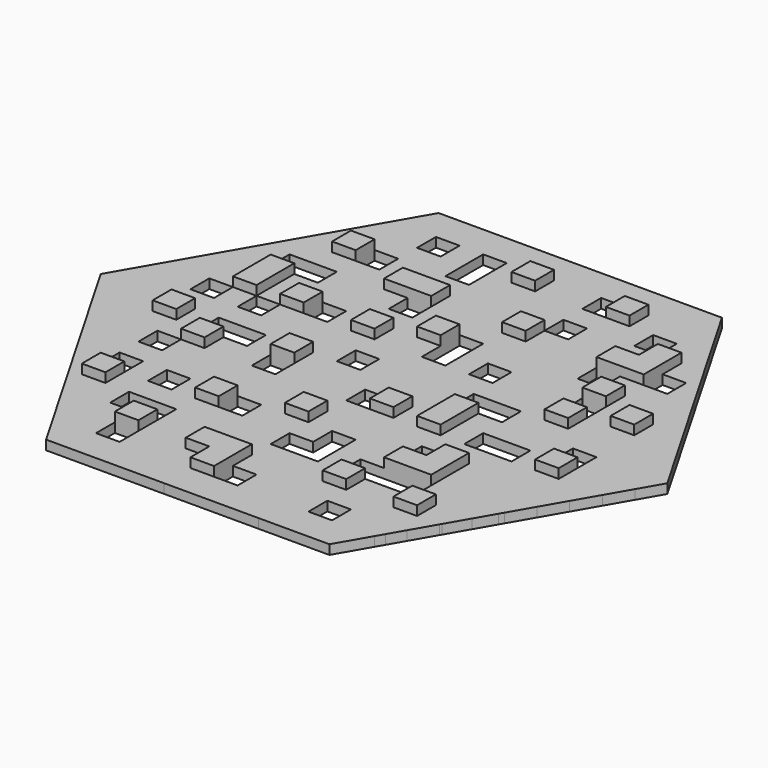
from build123d import *

# Parameters (mm, degrees)
F0_W     = 5
F0_H     = 5
F0_H_2   = 6.9615242271
F1_DEPTH = 2
F2_DEPTH = 4
F3_DEPTH = 25


with BuildPart() as f1:
    # F0 (on Top) → F1 (new body)
    with BuildSketch(Plane.XY):
        with Locations((27.5, 2.5)):
            Rectangle(F0_W, F0_H)
        with Locations((12.5, 12.5)):
            Rectangle(F0_W, F0_H)
        with Locations((7.5, 7.5)):
            Rectangle(F0_W, F0_H)
        with Locations((7.5, 12.5)):
            Rectangle(F0_W, F0_H)
        with Locations((-17.5, 27.5)):
            Rectangle(F0_W, F0_H)
        with Locations((12.5, 7.5)):
            Rectangle(F0_W, F0_H)
        with Locations((12.5, 32.5)):
            Rectangle(F0_W, F0_H)
        with Locations((2.5, -17.5)):
            Rectangle(F0_W, F0_H)
        with Locations((7.5, -37.5)):
            Rectangle(F0_W, F0_H)
        with Locations((12.5, -2.5)):
            Rectangle(F0_W, F0_H)
        with Locations((17.5, 12.5)):
            Rectangle(F0_W, F0_H)
        with Locations((-7.5, -27.5)):
            Rectangle(F0_W, F0_H)
        with Locations((7.5, -2.5)):
            Rectangle(F0_W, F0_H)
        with Locations((12.5, -7.5)):
            Rectangle(F0_W, F0_H)
        with Locations((-12.5, 42.5)):
            Rectangle(F0_W, F0_H)
        with Locations((-12.5, 7.5)):
            Rectangle(F0_W, F0_H)
        with Locations((2.5, 27.5)):
            Rectangle(F0_W, F0_H)
        with Locations((2.5, 37.5)):
            Rectangle(F0_W, F0_H)
        with Locations((2.5, -32.5)):
            Rectangle(F0_W, F0_H)
        with Locations((12.5, -17.5)):
            Rectangle(F0_W, F0_H)
        with Locations((-7.5, -7.5)):
            Rectangle(F0_W, F0_H)
        with Locations((-2.5, -12.5)):
            Rectangle(F0_W, F0_H)
        with Locations((-17.5, -2.5)):
            Rectangle(F0_W, F0_H)
        with Locations((17.5, 27.5)):
            Rectangle(F0_W, F0_H)
        with Locations((7.5, 22.5)):
            Rectangle(F0_W, F0_H)
        with Locations((-22.5, -22.5)):
            Rectangle(F0_W, F0_H)
        with Locations((2.5, 7.5)):
            Rectangle(F0_W, F0_H)
        with Locations((-7.5, -22.5)):
            Rectangle(F0_W, F0_H)
        with Locations((-2.5, -7.5)):
            Rectangle(F0_W, F0_H)
        with Locations((17.5, 42.5)):
            Rectangle(F0_W, F0_H)
        with Locations((12.5, -32.5)):
            Rectangle(F0_W, F0_H)
        with Locations((27.5, -22.5)):
            Rectangle(F0_W, F0_H)
        with Locations((22.5, 27.5)):
            Rectangle(F0_W, F0_H)
        with Locations((2.5, -22.5)):
            Rectangle(F0_W, F0_H)
        with Locations((-12.5, 17.5)):
            Rectangle(F0_W, F0_H)
        with Locations((22.5, -37.5)):
            Rectangle(F0_W, F0_H)
        with Locations((2.5, -7.5)):
            Rectangle(F0_W, F0_H)
        with Locations((27.5, 37.5)):
            Rectangle(F0_W, F0_H)
        with Locations((2.5, -12.5)):
            Rectangle(F0_W, F0_H)
        with Locations((-7.5, 17.5)):
            Rectangle(F0_W, F0_H)
        with Locations((27.5, 7.5)):
            Rectangle(F0_W, F0_H)
        with Locations((17.5, -32.5)):
            Rectangle(F0_W, F0_H)
        with Locations((-12.5, 2.5)):
            Rectangle(F0_W, F0_H)
        with Locations((27.5, -2.5)):
            Rectangle(F0_W, F0_H)
        with Locations((12.5, 42.5)):
            Rectangle(F0_W, F0_H)
        with Locations((22.5, -7.5)):
            Rectangle(F0_W, F0_H)
        with Locations((-7.5, 42.5)):
            Rectangle(F0_W, F0_H)
        with Locations((12.5, -22.5)):
            Rectangle(F0_W, F0_H)
        with Locations((-17.5, 22.5)):
            Rectangle(F0_W, F0_H)
        with Locations((17.5, 7.5)):
            Rectangle(F0_W, F0_H)
        with Locations((2.5, -27.5)):
            Rectangle(F0_W, F0_H)
        with Locations((2.5, 17.5)):
            Rectangle(F0_W, F0_H)
        with Locations((-2.5, -17.5)):
            Rectangle(F0_W, F0_H)
        with Locations((-22.5, -12.5)):
            Rectangle(F0_W, F0_H)
        with Locations((7.5, 27.5)):
            Rectangle(F0_W, F0_H)
        with Locations((7.5, 2.5)):
            Rectangle(F0_W, F0_H)
        with Locations((17.5, -27.5)):
            Rectangle(F0_W, F0_H)
        with Locations((-12.5, -27.5)):
            Rectangle(F0_W, F0_H)
        with Locations((17.5, -22.5)):
            Rectangle(F0_W, F0_H)
        with Locations((22.5, 17.5)):
            Rectangle(F0_W, F0_H)
        with Locations((7.5, -12.5)):
            Rectangle(F0_W, F0_H)
        with Locations((-2.5, 27.5)):
            Rectangle(F0_W, F0_H)
        with Locations((-2.5, -2.5)):
            Rectangle(F0_W, F0_H)
        with Locations((17.5, -2.5)):
            Rectangle(F0_W, F0_H)
        with Locations((-22.5, 7.5)):
            Rectangle(F0_W, F0_H)
        with Locations((-2.5, -37.5)):
            Rectangle(F0_W, F0_H)
        with Locations((-17.5, 7.5)):
            Rectangle(F0_W, F0_H)
        with Locations((-22.5, 22.5)):
            Rectangle(F0_W, F0_H)
        with Locations((17.5, 22.5)):
            Rectangle(F0_W, F0_H)
        with Locations((-7.5, -37.5)):
            Rectangle(F0_W, F0_H)
        with Locations((-17.5, -7.5)):
            Rectangle(F0_W, F0_H)
        with Locations((-2.5, -22.5)):
            Rectangle(F0_W, F0_H)
        with Locations((22.5, -22.5)):
            Rectangle(F0_W, F0_H)
        with Locations((-12.5, -22.5)):
            Rectangle(F0_W, F0_H)
        with Locations((-2.5, 2.5)):
            Rectangle(F0_W, F0_H)
        with Locations((-22.5, -37.5)):
            Rectangle(F0_W, F0_H)
        with Locations((27.5, 27.5)):
            Rectangle(F0_W, F0_H)
        with Locations((-2.5, 17.5)):
            Rectangle(F0_W, F0_H)
        with Locations((-12.5, -2.5)):
            Rectangle(F0_W, F0_H)
        with Locations((-22.5, 17.5)):
            Rectangle(F0_W, F0_H)
        with Locations((-7.5, -17.5)):
            Rectangle(F0_W, F0_H)
        with Locations((7.5, -17.5)):
            Rectangle(F0_W, F0_H)
        with Locations((27.5, -27.5)):
            Rectangle(F0_W, F0_H)
        with Locations((-12.5, -32.5)):
            Rectangle(F0_W, F0_H)
        with Locations((-22.5, -7.5)):
            Rectangle(F0_W, F0_H)
        with Locations((-7.5, -2.5)):
            Rectangle(F0_W, F0_H)
        with Locations((12.5, -12.5)):
            Rectangle(F0_W, F0_H)
        with Locations((-17.5, -32.5)):
            Rectangle(F0_W, F0_H)
        with Locations((22.5, -27.5)):
            Rectangle(F0_W, F0_H)
        with Locations((12.5, -37.5)):
            Rectangle(F0_W, F0_H)
        with Locations((-17.5, -17.5)):
            Rectangle(F0_W, F0_H)
        with Locations((17.5, -17.5)):
            Rectangle(F0_W, F0_H)
        with Locations((-12.5, -37.5)):
            Rectangle(F0_W, F0_H)
        with Locations((-17.5, -27.5)):
            Rectangle(F0_W, F0_H)
        with Locations((2.5, 2.5)):
            Rectangle(F0_W, F0_H)
        with Locations((-22.5, -17.5)):
            Rectangle(F0_W, F0_H)
        with Locations((-2.5, 32.5)):
            Rectangle(F0_W, F0_H)
        with Locations((-17.5, 2.5)):
            Rectangle(F0_W, F0_H)
        with Locations((2.5, 12.5)):
            Rectangle(F0_W, F0_H)
        with Locations((12.5, 2.5)):
            Rectangle(F0_W, F0_H)
        with Locations((12.5, -27.5)):
            Rectangle(F0_W, F0_H)
        with Locations((22.5, 42.5)):
            Rectangle(F0_W, F0_H)
        with Locations((-22.5, 32.5)):
            Rectangle(F0_W, F0_H)
        with Locations((2.5, -2.5)):
            Rectangle(F0_W, F0_H)
        with Locations((-7.5, 2.5)):
            Rectangle(F0_W, F0_H)
        with Locations((-2.5, 12.5)):
            Rectangle(F0_W, F0_H)
        with Locations((-2.5, -32.5)):
            Rectangle(F0_W, F0_H)
        with Locations((27.5, -37.5)):
            Rectangle(F0_W, F0_H)
        with Locations((-17.5, 32.5)):
            Rectangle(F0_W, F0_H)
        with Locations((-12.5, -17.5)):
            Rectangle(F0_W, F0_H)
        with Locations((7.5, 32.5)):
            Rectangle(F0_W, F0_H)
        with Locations((22.5, -32.5)):
            Rectangle(F0_W, F0_H)
        with Locations((2.5, 32.5)):
            Rectangle(F0_W, F0_H)
        with Locations((-7.5, 7.5)):
            Rectangle(F0_W, F0_H)
        with Locations((17.5, -12.5)):
            Rectangle(F0_W, F0_H)
        with Locations((27.5, 17.5)):
            Rectangle(F0_W, F0_H)
        with Locations((-22.5, -32.5)):
            Rectangle(F0_W, F0_H)
        with Locations((-12.5, 32.5)):
            Rectangle(F0_W, F0_H)
        with Locations((7.5, -27.5)):
            Rectangle(F0_W, F0_H)
        with Locations((-7.5, 32.5)):
            Rectangle(F0_W, F0_H)
        with Locations((7.5, 42.5)):
            Rectangle(F0_W, F0_H)
        with Locations((-7.5, 22.5)):
            Rectangle(F0_W, F0_H)
        with Locations((-12.5, 27.5)):
            Rectangle(F0_W, F0_H)
        with Locations((27.5, -12.5)):
            Rectangle(F0_W, F0_H)
        with Locations((27.5, -32.5)):
            Rectangle(F0_W, F0_H)
        with Locations((-17.5, -22.5)):
            Rectangle(F0_W, F0_H)
        with Locations((7.5, -22.5)):
            Rectangle(F0_W, F0_H)
        with Locations((-22.5, 12.5)):
            Rectangle(F0_W, F0_H)
        with Locations((22.5, -17.5)):
            Rectangle(F0_W, F0_H)
        with Locations((17.5, -7.5)):
            Rectangle(F0_W, F0_H)
        with Locations((-22.5, 42.5)):
            Rectangle(F0_W, F0_H)
        with Locations((27.5, 22.5)):
            Rectangle(F0_W, F0_H)
        with Locations((22.5, -2.5)):
            Rectangle(F0_W, F0_H)
        with Locations((-2.5, 7.5)):
            Rectangle(F0_W, F0_H)
        with Locations((-2.5, -27.5)):
            Rectangle(F0_W, F0_H)
        with Locations((17.5, 17.5)):
            Rectangle(F0_W, F0_H)
        with Locations((27.5, 32.5)):
            Rectangle(F0_W, F0_H)
        with Locations((12.5, 22.5)):
            Rectangle(F0_W, F0_H)
        with Locations((2.5, 42.5)):
            Rectangle(F0_W, F0_H)
        with Locations((22.5, -12.5)):
            Rectangle(F0_W, F0_H)
        with Locations((22.5, 22.5)):
            Rectangle(F0_W, F0_H)
        with Locations((-7.5, 27.5)):
            Rectangle(F0_W, F0_H)
        with Locations((-12.5, -7.5)):
            Rectangle(F0_W, F0_H)
        with Locations((-12.5, 22.5)):
            Rectangle(F0_W, F0_H)
        with Locations((-17.5, 17.5)):
            Rectangle(F0_W, F0_H)
        with Locations((-17.5, 12.5)):
            Rectangle(F0_W, F0_H)
        with Locations((27.5, -7.5)):
            Rectangle(F0_W, F0_H)
        with Locations((-7.5, -32.5)):
            Rectangle(F0_W, F0_H)
        with Locations((17.5, 37.5)):
            Rectangle(F0_W, F0_H)
        with Locations((12.5, 17.5)):
            Rectangle(F0_W, F0_H)
        with Locations((-12.5, 37.5)):
            Rectangle(F0_W, F0_H)
        with Locations((-7.5, 12.5)):
            Rectangle(F0_W, F0_H)
        with Locations((-2.5, 37.5)):
            Rectangle(F0_W, F0_H)
        with Locations((22.5, 2.5)):
            Rectangle(F0_W, F0_H)
        with Locations((-22.5, -2.5)):
            Rectangle(F0_W, F0_H)
        with Locations((-2.5, 42.5)):
            Rectangle(F0_W, F0_H)
        with Locations((17.5, 2.5)):
            Rectangle(F0_W, F0_H)
        with Locations((27.5, 42.5)):
            Rectangle(F0_W, F0_H)
        with Locations((27.5, 12.5)):
            Rectangle(F0_W, F0_H)
        with Locations((-12.5, 12.5)):
            Rectangle(F0_W, F0_H)
        with Locations((-22.5, 37.5)):
            Rectangle(F0_W, F0_H)
        with Locations((17.5, 32.5)):
            Rectangle(F0_W, F0_H)
        with Locations((7.5, 37.5)):
            Rectangle(F0_W, F0_H)
        with Locations((22.5, 12.5)):
            Rectangle(F0_W, F0_H)
        with Locations((-2.5, 22.5)):
            Rectangle(F0_W, F0_H)
        with Locations((2.5, -37.5)):
            Rectangle(F0_W, F0_H)
        with Locations((27.5, -17.5)):
            Rectangle(F0_W, F0_H)
        with Locations((7.5, -32.5)):
            Rectangle(F0_W, F0_H)
        with Locations((-7.5, 37.5)):
            Rectangle(F0_W, F0_H)
        with Locations((-17.5, -37.5)):
            Rectangle(F0_W, F0_H)
        with Locations((17.5, -37.5)):
            Rectangle(F0_W, F0_H)
        with Locations((22.5, 37.5)):
            Rectangle(F0_W, F0_H)
        with Locations((7.5, 17.5)):
            Rectangle(F0_W, F0_H)
        with Locations((-7.5, -12.5)):
            Rectangle(F0_W, F0_H)
        with Locations((12.5, 27.5)):
            Rectangle(F0_W, F0_H)
        with Locations((-17.5, -12.5)):
            Rectangle(F0_W, F0_H)
        with Locations((-22.5, -27.5)):
            Rectangle(F0_W, F0_H)
        with Locations((22.5, 7.5)):
            Rectangle(F0_W, F0_H)
        with Locations((2.5, 22.5)):
            Rectangle(F0_W, F0_H)
        with Locations((-12.5, -12.5)):
            Rectangle(F0_W, F0_H)
        with Locations((12.5, 37.5)):
            Rectangle(F0_W, F0_H)
        with Locations((7.5, -7.5)):
            Rectangle(F0_W, F0_H)
        with Locations((22.5, 32.5)):
            Rectangle(F0_W, F0_H)
        with Locations((-17.5, 37.5)):
            Rectangle(F0_W, F0_H)
        with Locations((-22.5, 27.5)):
            Rectangle(F0_W, F0_H)
        with Locations((-17.5, 42.5)):
            Rectangle(F0_W, F0_H)
        with Locations((-22.5, 2.5)):
            Rectangle(F0_W, F0_H)
        with Locations((-27.5, 42.5)):
            Rectangle(F0_W, F0_H)
        with Locations((-27.5, 37.5)):
            Rectangle(F0_W, F0_H)
        with Locations((-27.5, 32.5)):
            Rectangle(F0_W, F0_H)
        with Locations((-27.5, 27.5)):
            Rectangle(F0_W, F0_H)
        with Locations((-27.5, 22.5)):
            Rectangle(F0_W, F0_H)
        with Locations((-27.5, 17.5)):
            Rectangle(F0_W, F0_H)
        with Locations((-27.5, 12.5)):
            Rectangle(F0_W, F0_H)
        with Locations((-27.5, 7.5)):
            Rectangle(F0_W, F0_H)
        with Locations((-27.5, 2.5)):
            Rectangle(F0_W, F0_H)
        with Locations((-27.5, -2.5)):
            Rectangle(F0_W, F0_H)
        with Locations((-27.5, -7.5)):
            Rectangle(F0_W, F0_H)
        with Locations((-27.5, -12.5)):
            Rectangle(F0_W, F0_H)
        with Locations((-27.5, -17.5)):
            Rectangle(F0_W, F0_H)
        with Locations((-27.5, -22.5)):
            Rectangle(F0_W, F0_H)
        with Locations((-27.5, -27.5)):
            Rectangle(F0_W, F0_H)
        with Locations((-27.5, -32.5)):
            Rectangle(F0_W, F0_H)
        with Locations((-27.5, -37.5)):
            Rectangle(F0_W, F0_H)
        with Locations((-32.5, -37.5)):
            Rectangle(F0_W, F0_H)
        with Locations((-32.5, -32.5)):
            Rectangle(F0_W, F0_H)
        with Locations((-32.5, -27.5)):
            Rectangle(F0_W, F0_H)
        with Locations((-32.5, -22.5)):
            Rectangle(F0_W, F0_H)
        with Locations((-32.5, -17.5)):
            Rectangle(F0_W, F0_H)
        with Locations((-32.5, -12.5)):
            Rectangle(F0_W, F0_H)
        with Locations((-32.5, -7.5)):
            Rectangle(F0_W, F0_H)
        with Locations((-32.5, -2.5)):
            Rectangle(F0_W, F0_H)
        with Locations((-32.5, 2.5)):
            Rectangle(F0_W, F0_H)
        with Locations((-32.5, 7.5)):
            Rectangle(F0_W, F0_H)
        with Locations((-32.5, 12.5)):
            Rectangle(F0_W, F0_H)
        with Locations((-32.5, 17.5)):
            Rectangle(F0_W, F0_H)
        with Locations((-32.5, 22.5)):
            Rectangle(F0_W, F0_H)
        with Locations((-32.5, 27.5)):
            Rectangle(F0_W, F0_H)
        with Locations((-32.5, 32.5)):
            Rectangle(F0_W, F0_H)
        with Locations((-32.5, 37.5)):
            Rectangle(F0_W, F0_H)
        Polygon((-34.0192378865, 45), (-35, 43.3012701892), (-35, 40), (-30, 40), (-30, 45), align=None)
        Polygon((-30, 51.9615242271), (-34.0192378865, 45), (-30, 45), align=None)
        with Locations((-27.5, 48.4807621135)):
            Rectangle(F0_W, F0_H_2)
        with Locations((-22.5, 48.4807621135)):
            Rectangle(F0_W, F0_H_2)
        Polygon((45, 5), (45, 0), (60, 0), (57.1132486541, 5), align=None)
        Polygon((45, 25), (45, 20), (48.4529946162, 20), (45.5662432703, 25), align=None)
        with Locations((-37.5, 2.5)):
            Rectangle(F0_W, F0_H)
        with Locations((17.5, -48.4807621135)):
            Rectangle(F0_W, F0_H_2)
        with Locations((42.5, 12.5)):
            Rectangle(F0_W, F0_H)
        with Locations((42.5, -22.5)):
            Rectangle(F0_W, F0_H)
        with Locations((32.5, 12.5)):
            Rectangle(F0_W, F0_H)
        Polygon((40, -30), (35, -30), (35, -35), (39.7927405784, -35), (40, -34.6410161514), align=None)
        with Locations((17.5, -42.5)):
            Rectangle(F0_W, F0_H)
        with Locations((-37.5, -22.5)):
            Rectangle(F0_W, F0_H)
        with Locations((2.5, -42.5)):
            Rectangle(F0_W, F0_H)
        with Locations((37.5, 27.5)):
            Rectangle(F0_W, F0_H)
        with Locations((32.5, -2.5)):
            Rectangle(F0_W, F0_H)
        with Locations((42.5, 7.5)):
            Rectangle(F0_W, F0_H)
        Polygon((-45.5662432703, 25), (-48.4529946162, 20), (-45, 20), (-45, 25), align=None)
        with Locations((-12.5, -48.4807621135)):
            Rectangle(F0_W, F0_H_2)
        with Locations((-17.5, -42.5)):
            Rectangle(F0_W, F0_H)
        Polygon((-40, 34.6410161514), (-42.6794919243, 30), (-40, 30), align=None)
        with Locations((-42.5, 22.5)):
            Rectangle(F0_W, F0_H)
        with Locations((-42.5, -2.5)):
            Rectangle(F0_W, F0_H)
        with Locations((32.5, 27.5)):
            Rectangle(F0_W, F0_H)
        with Locations((42.5, -17.5)):
            Rectangle(F0_W, F0_H)
        with Locations((32.5, -32.5)):
            Rectangle(F0_W, F0_H)
        with Locations((32.5, -37.5)):
            Rectangle(F0_W, F0_H)
        with Locations((-27.5, -42.5)):
            Rectangle(F0_W, F0_H)
        with Locations((32.5, 22.5)):
            Rectangle(F0_W, F0_H)
        with Locations((-27.5, -48.4807621135)):
            Rectangle(F0_W, F0_H_2)
        Polygon((35, 40), (35, 35), (39.7927405784, 35), (36.9059892324, 40), align=None)
        Polygon((-30, -45), (-34.0192378865, -45), (-30, -51.9615242271), align=None)
        with Locations((-37.5, -7.5)):
            Rectangle(F0_W, F0_H)
        with Locations((32.5, -17.5)):
            Rectangle(F0_W, F0_H)
        with Locations((-22.5, -42.5)):
            Rectangle(F0_W, F0_H)
        with Locations((17.5, 48.4807621135)):
            Rectangle(F0_W, F0_H_2)
        with Locations((-17.5, -48.4807621135)):
            Rectangle(F0_W, F0_H_2)
        with Locations((32.5, 2.5)):
            Rectangle(F0_W, F0_H)
        Polygon((45, 15), (45, 10), (54.2264973081, 10), (51.3397459622, 15), align=None)
        with Locations((-37.5, -2.5)):
            Rectangle(F0_W, F0_H)
        with Locations((-42.5, -12.5)):
            Rectangle(F0_W, F0_H)
        with Locations((7.5, -42.5)):
            Rectangle(F0_W, F0_H)
        with Locations((27.5, 48.4807621135)):
            Rectangle(F0_W, F0_H_2)
        with Locations((-42.5, 7.5)):
            Rectangle(F0_W, F0_H)
        with Locations((37.5, 22.5)):
            Rectangle(F0_W, F0_H)
        Polygon((51.3397459622, -15), (45, -15), (45, -20), (48.4529946162, -20), align=None)
        Polygon((-45, -10), (-54.2264973081, -10), (-51.3397459622, -15), (-45, -15), align=None)
        with Locations((-42.5, -22.5)):
            Rectangle(F0_W, F0_H)
        with Locations((42.5, -7.5)):
            Rectangle(F0_W, F0_H)
        Polygon((40, 34.6410161514), (40, 30), (42.6794919243, 30), align=None)
        with Locations((32.5, 17.5)):
            Rectangle(F0_W, F0_H)
        with Locations((-37.5, 27.5)):
            Rectangle(F0_W, F0_H)
        Polygon((-39.7927405784, 35), (-40, 34.6410161514), (-40, 30), (-35, 30), (-35, 35), align=None)
        Polygon((-45, -25), (-45, -25.9807621135), (-42.6794919243, -30), (-40, -30), (-40, -25), align=None)
        with Locations((2.5, -48.4807621135)):
            Rectangle(F0_W, F0_H_2)
        with Locations((-42.5, 12.5)):
            Rectangle(F0_W, F0_H)
        with Locations((-42.5, 17.5)):
            Rectangle(F0_W, F0_H)
        with Locations((37.5, 7.5)):
            Rectangle(F0_W, F0_H)
        with Locations((37.5, -7.5)):
            Rectangle(F0_W, F0_H)
        with Locations((-37.5, -12.5)):
            Rectangle(F0_W, F0_H)
        with Locations((32.5, -7.5)):
            Rectangle(F0_W, F0_H)
        Polygon((-48.4529946162, 20), (-51.3397459622, 15), (-45, 15), (-45, 20), align=None)
        with Locations((37.5, -27.5)):
            Rectangle(F0_W, F0_H)
        with Locations((-37.5, -17.5)):
            Rectangle(F0_W, F0_H)
        with Locations((7.5, -48.4807621135)):
            Rectangle(F0_W, F0_H_2)
        Polygon((-42.6794919243, 30), (-45, 25.9807621135), (-45, 25), (-40, 25), (-40, 30), align=None)
        Polygon((-35, -40), (-35, -43.3012701892), (-34.0192378865, -45), (-30, -45), (-30, -40), align=None)
        Polygon((57.1132486541, -5), (45, -5), (45, -10), (54.2264973081, -10), align=None)
        Polygon((40, 30), (40, 25), (45, 25), (45, 25.9807621135), (42.6794919243, 30), align=None)
        with Locations((-17.5, 48.4807621135)):
            Rectangle(F0_W, F0_H_2)
        with Locations((32.5, -12.5)):
            Rectangle(F0_W, F0_H)
        Polygon((54.2264973081, -10), (45, -10), (45, -15), (51.3397459622, -15), align=None)
        with Locations((32.5, 32.5)):
            Rectangle(F0_W, F0_H)
        Polygon((48.4529946162, -20), (45, -20), (45, -25), (45.5662432703, -25), align=None)
        Polygon((42.6794919243, -30), (40, -30), (40, -34.6410161514), align=None)
        Polygon((45, 20), (45, 15), (51.3397459622, 15), (48.4529946162, 20), align=None)
        Polygon((-35, -35), (-39.7927405784, -35), (-36.9059892324, -40), (-35, -40), align=None)
        with Locations((37.5, 2.5)):
            Rectangle(F0_W, F0_H)
        with Locations((32.5, -22.5)):
            Rectangle(F0_W, F0_H)
        Polygon((34.0192378865, 45), (30, 51.9615242271), (30, 45), align=None)
        with Locations((12.5, -42.5)):
            Rectangle(F0_W, F0_H)
        with Locations((-7.5, 48.4807621135)):
            Rectangle(F0_W, F0_H_2)
        with Locations((-7.5, -48.4807621135)):
            Rectangle(F0_W, F0_H_2)
        Polygon((-40, -30), (-42.6794919243, -30), (-40, -34.6410161514), align=None)
        Polygon((35, 43.3012701892), (35, 40), (36.9059892324, 40), align=None)
        with Locations((2.5, 48.4807621135)):
            Rectangle(F0_W, F0_H_2)
        with Locations((37.5, 12.5)):
            Rectangle(F0_W, F0_H)
        with Locations((22.5, -48.4807621135)):
            Rectangle(F0_W, F0_H_2)
        with Locations((42.5, -2.5)):
            Rectangle(F0_W, F0_H)
        with Locations((-37.5, 7.5)):
            Rectangle(F0_W, F0_H)
        with Locations((32.5, 37.5)):
            Rectangle(F0_W, F0_H)
        with Locations((-37.5, -27.5)):
            Rectangle(F0_W, F0_H)
        Polygon((35, 35), (35, 30), (40, 30), (40, 34.6410161514), (39.7927405784, 35), align=None)
        with Locations((-7.5, -42.5)):
            Rectangle(F0_W, F0_H)
        Polygon((-40, -30), (-40, -34.6410161514), (-39.7927405784, -35), (-35, -35), (-35, -30), align=None)
        with Locations((37.5, -12.5)):
            Rectangle(F0_W, F0_H)
        with Locations((37.5, -2.5)):
            Rectangle(F0_W, F0_H)
        with Locations((-22.5, -48.4807621135)):
            Rectangle(F0_W, F0_H_2)
        Polygon((-35, 43.3012701892), (-36.9059892324, 40), (-35, 40), align=None)
        Polygon((-51.3397459622, 15), (-54.2264973081, 10), (-45, 10), (-45, 15), align=None)
        Polygon((30, -45), (30, -51.9615242271), (34.0192378865, -45), align=None)
        Polygon((35, -40), (30, -40), (30, -45), (34.0192378865, -45), (35, -43.3012701892), align=None)
        Polygon((39.7927405784, -35), (35, -35), (35, -40), (36.9059892324, -40), align=None)
        with Locations((22.5, -42.5)):
            Rectangle(F0_W, F0_H)
        with Locations((32.5, -27.5)):
            Rectangle(F0_W, F0_H)
        with Locations((-2.5, 48.4807621135)):
            Rectangle(F0_W, F0_H_2)
        with Locations((7.5, 48.4807621135)):
            Rectangle(F0_W, F0_H_2)
        with Locations((37.5, -22.5)):
            Rectangle(F0_W, F0_H)
        with Locations((42.5, 17.5)):
            Rectangle(F0_W, F0_H)
        with Locations((32.5, 7.5)):
            Rectangle(F0_W, F0_H)
        with Locations((42.5, -12.5)):
            Rectangle(F0_W, F0_H)
        Polygon((-36.9059892324, 40), (-39.7927405784, 35), (-35, 35), (-35, 40), align=None)
        with Locations((-2.5, -42.5)):
            Rectangle(F0_W, F0_H)
        with Locations((-37.5, 17.5)):
            Rectangle(F0_W, F0_H)
        Polygon((30, 45), (30, 40), (35, 40), (35, 43.3012701892), (34.0192378865, 45), align=None)
        with Locations((12.5, 48.4807621135)):
            Rectangle(F0_W, F0_H_2)
        Polygon((45, -25), (40, -25), (40, -30), (42.6794919243, -30), (45, -25.9807621135), align=None)
        with Locations((27.5, -42.5)):
            Rectangle(F0_W, F0_H)
        with Locations((-12.5, 48.4807621135)):
            Rectangle(F0_W, F0_H_2)
        Polygon((60, 0), (45, 0), (45, -5), (57.1132486541, -5), align=None)
        with Locations((22.5, 48.4807621135)):
            Rectangle(F0_W, F0_H_2)
        with Locations((-42.5, -7.5)):
            Rectangle(F0_W, F0_H)
        with Locations((-12.5, -42.5)):
            Rectangle(F0_W, F0_H)
        with Locations((-2.5, -48.4807621135)):
            Rectangle(F0_W, F0_H_2)
        Polygon((45, 10), (45, 5), (57.1132486541, 5), (54.2264973081, 10), align=None)
        with Locations((-37.5, 22.5)):
            Rectangle(F0_W, F0_H)
        with Locations((37.5, 17.5)):
            Rectangle(F0_W, F0_H)
        with Locations((-42.5, -17.5)):
            Rectangle(F0_W, F0_H)
        Polygon((-45, -15), (-51.3397459622, -15), (-48.4529946162, -20), (-45, -20), align=None)
        with Locations((-42.5, 2.5)):
            Rectangle(F0_W, F0_H)
        with Locations((27.5, -48.4807621135)):
            Rectangle(F0_W, F0_H_2)
        with Locations((42.5, 22.5)):
            Rectangle(F0_W, F0_H)
        Polygon((-45, -20), (-48.4529946162, -20), (-45.5662432703, -25), (-45, -25), align=None)
        with Locations((42.5, 2.5)):
            Rectangle(F0_W, F0_H)
        with Locations((37.5, -17.5)):
            Rectangle(F0_W, F0_H)
        with Locations((12.5, -48.4807621135)):
            Rectangle(F0_W, F0_H_2)
        with Locations((-37.5, 12.5)):
            Rectangle(F0_W, F0_H)
        Polygon((-45, 25.9807621135), (-45.5662432703, 25), (-45, 25), align=None)
        Polygon((45.5662432703, -25), (45, -25), (45, -25.9807621135), align=None)
        Polygon((45, 25.9807621135), (45, 25), (45.5662432703, 25), align=None)
        Polygon((36.9059892324, -40), (35, -40), (35, -43.3012701892), align=None)
        Polygon((-35, -40), (-36.9059892324, -40), (-35, -43.3012701892), align=None)
        Polygon((-45, -25), (-45.5662432703, -25), (-45, -25.9807621135), align=None)
        Polygon((-54.2264973081, 10), (-57.1132486541, 5), (-45, 5), (-45, 10), align=None)
        Polygon((-57.1132486541, 5), (-60, 0), (-45, 0), (-45, 5), align=None)
        Polygon((-45, 0), (-60, 0), (-57.1132486541, -5), (-45, -5), align=None)
        Polygon((-45, -5), (-57.1132486541, -5), (-54.2264973081, -10), (-45, -10), align=None)
    extrude(amount=F1_DEPTH)

    # F0 (on Top) → F2 (join)
    with BuildSketch(Plane.XY):
        with Locations((-12.5, 12.5)):
            Rectangle(F0_W, F0_H)
        with Locations((-2.5, 17.5)):
            Rectangle(F0_W, F0_H)
        with Locations((7.5, 27.5)):
            Rectangle(F0_W, F0_H)
        with Locations((-2.5, -17.5)):
            Rectangle(F0_W, F0_H)
        with Locations((-17.5, -22.5)):
            Rectangle(F0_W, F0_H)
        with Locations((-32.5, -7.5)):
            Rectangle(F0_W, F0_H)
        with Locations((-22.5, -37.5)):
            Rectangle(F0_W, F0_H)
        with Locations((-42.5, -2.5)):
            Rectangle(F0_W, F0_H)
        with Locations((-37.5, 12.5)):
            Rectangle(F0_W, F0_H)
        with Locations((-37.5, 17.5)):
            Rectangle(F0_W, F0_H)
        with Locations((-32.5, 32.5)):
            Rectangle(F0_W, F0_H)
        with Locations((-22.5, 42.5)):
            Rectangle(F0_W, F0_H)
        with Locations((17.5, 42.5)):
            Rectangle(F0_W, F0_H)
        with Locations((12.5, 42.5)):
            Rectangle(F0_W, F0_H)
        with Locations((27.5, 27.5)):
            Rectangle(F0_W, F0_H)
        with Locations((32.5, 32.5)):
            Rectangle(F0_W, F0_H)
        with Locations((32.5, 17.5)):
            Rectangle(F0_W, F0_H)
        with Locations((32.5, 7.5)):
            Rectangle(F0_W, F0_H)
        with Locations((42.5, 12.5)):
            Rectangle(F0_W, F0_H)
        with Locations((42.5, -7.5)):
            Rectangle(F0_W, F0_H)
        with Locations((22.5, -22.5)):
            Rectangle(F0_W, F0_H)
        with Locations((17.5, -32.5)):
            Rectangle(F0_W, F0_H)
        with Locations((32.5, 27.5)):
            Rectangle(F0_W, F0_H)
        with Locations((-12.5, 27.5)):
            Rectangle(F0_W, F0_H)
        with Locations((-17.5, 27.5)):
            Rectangle(F0_W, F0_H)
        with Locations((-17.5, -2.5)):
            Rectangle(F0_W, F0_H)
        with Locations((-27.5, 12.5)):
            Rectangle(F0_W, F0_H)
        with Locations((-7.5, -37.5)):
            Rectangle(F0_W, F0_H)
        with Locations((32.5, -32.5)):
            Rectangle(F0_W, F0_H)
        with Locations((17.5, -2.5)):
            Rectangle(F0_W, F0_H)
        with Locations((17.5, -7.5)):
            Rectangle(F0_W, F0_H)
        with Locations((7.5, -7.5)):
            Rectangle(F0_W, F0_H)
        with Locations((12.5, 12.5)):
            Rectangle(F0_W, F0_H)
        with Locations((-2.5, 42.5)):
            Rectangle(F0_W, F0_H)
        with Locations((-37.5, -27.5)):
            Rectangle(F0_W, F0_H)
        with Locations((-2.5, -42.5)):
            Rectangle(F0_W, F0_H)
        with Locations((27.5, -17.5)):
            Rectangle(F0_W, F0_H)
        with Locations((-2.5, -37.5)):
            Rectangle(F0_W, F0_H)
        with Locations((22.5, -42.5)):
            Rectangle(F0_W, F0_H)
        with Locations((27.5, -22.5)):
            Rectangle(F0_W, F0_H)
        with Locations((7.5, -27.5)):
            Rectangle(F0_W, F0_H)
    extrude(amount=F2_DEPTH)

    # F0 (on Top) → F3 (cut)
    with BuildSketch(Plane.XY):
        with Locations((-12.5, -22.5)):
            Rectangle(F0_W, F0_H)
        with Locations((2.5, -27.5)):
            Rectangle(F0_W, F0_H)
        with Locations((7.5, -22.5)):
            Rectangle(F0_W, F0_H)
        with Locations((7.5, -27.5)):
            Rectangle(F0_W, F0_H)
        with Locations((22.5, -27.5)):
            Rectangle(F0_W, F0_H)
        with Locations((22.5, -42.5)):
            Rectangle(F0_W, F0_H)
        with Locations((-27.5, -32.5)):
            Rectangle(F0_W, F0_H)
        with Locations((-22.5, -32.5)):
            Rectangle(F0_W, F0_H)
        with Locations((-27.5, -22.5)):
            Rectangle(F0_W, F0_H)
        with Locations((-37.5, -22.5)):
            Rectangle(F0_W, F0_H)
        with Locations((-37.5, -12.5)):
            Rectangle(F0_W, F0_H)
        with Locations((-17.5, -7.5)):
            Rectangle(F0_W, F0_H)
        with Locations((-27.5, -2.5)):
            Rectangle(F0_W, F0_H)
        with Locations((-32.5, 7.5)):
            Rectangle(F0_W, F0_H)
        with Locations((-42.5, 7.5)):
            Rectangle(F0_W, F0_H)
        with Locations((-37.5, 22.5)):
            Rectangle(F0_W, F0_H)
        with Locations((-32.5, 22.5)):
            Rectangle(F0_W, F0_H)
        with Locations((-27.5, 32.5)):
            Rectangle(F0_W, F0_H)
        with Locations((-22.5, 42.5)):
            Rectangle(F0_W, F0_H)
        with Locations((-12.5, 42.5)):
            Rectangle(F0_W, F0_H)
        with Locations((-12.5, 37.5)):
            Rectangle(F0_W, F0_H)
        with Locations((-12.5, 22.5)):
            Rectangle(F0_W, F0_H)
        with Locations((-22.5, 12.5)):
            Rectangle(F0_W, F0_H)
        with Locations((-7.5, 2.5)):
            Rectangle(F0_W, F0_H)
        with Locations((12.5, 12.5)):
            Rectangle(F0_W, F0_H)
        with Locations((2.5, 17.5)):
            Rectangle(F0_W, F0_H)
        with Locations((12.5, 32.5)):
            Rectangle(F0_W, F0_H)
        with Locations((12.5, 42.5)):
            Rectangle(F0_W, F0_H)
        with Locations((27.5, 37.5)):
            Rectangle(F0_W, F0_H)
        with Locations((37.5, 27.5)):
            Rectangle(F0_W, F0_H)
        with Locations((27.5, 22.5)):
            Rectangle(F0_W, F0_H)
        with Locations((32.5, 12.5)):
            Rectangle(F0_W, F0_H)
        with Locations((22.5, 2.5)):
            Rectangle(F0_W, F0_H)
        with Locations((27.5, -7.5)):
            Rectangle(F0_W, F0_H)
        with Locations((22.5, -17.5)):
            Rectangle(F0_W, F0_H)
        with Locations((27.5, -27.5)):
            Rectangle(F0_W, F0_H)
        with Locations((2.5, -42.5)):
            Rectangle(F0_W, F0_H)
        with Locations((32.5, -7.5)):
            Rectangle(F0_W, F0_H)
        with Locations((42.5, -2.5)):
            Rectangle(F0_W, F0_H)
        with Locations((2.5, -7.5)):
            Rectangle(F0_W, F0_H)
        with Locations((2.5, 12.5)):
            Rectangle(F0_W, F0_H)
        with Locations((-32.5, -2.5)):
            Rectangle(F0_W, F0_H)
        with Locations((17.5, 2.5)):
            Rectangle(F0_W, F0_H)
        with Locations((-22.5, -42.5)):
            Rectangle(F0_W, F0_H)
        with Locations((17.5, -27.5)):
            Rectangle(F0_W, F0_H)
    extrude(amount=F3_DEPTH, mode=Mode.SUBTRACT)


solid = f1.part
